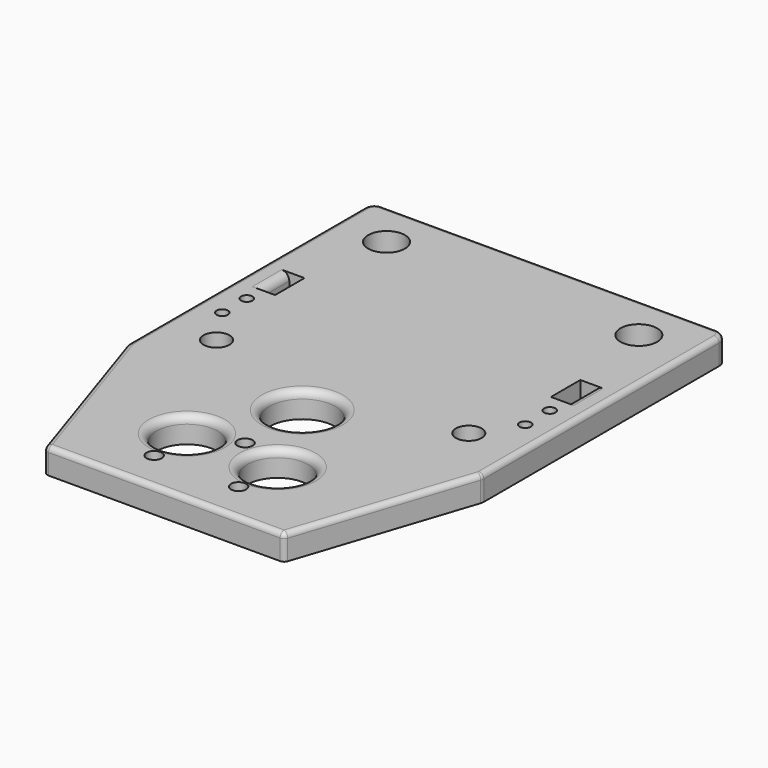
from build123d import *

# Parameters (mm, degrees)
F0_R     = 1.5
F0_R_2   = 6
F0_R_3   = 2.55
F0_R_4   = 6.5
F0_R_5   = 1.125
F0_W     = 3
F0_H     = 7.25
F0_R_6   = 3.625
F1_DEPTH = 5
F2_R     = 1.5
F3_R     = 1.5
F4_SIZE  = 1.5
F5_SIZE  = 1.5
F7_R     = 1


# Not quite as in the source:
# - a fillet or chamfer that OpenCascade refuses, or shapes differently, is made with other operations: its cross-section is extruded or revolved along the edge and cut away or added


with BuildPart() as f1:
    # F0 (on Top) → F1 (new body)
    with BuildSketch(Plane.XY):
        with BuildLine():
            Line((33, 31.9801117687), (0, 31.9801117687))
            Line((0, 31.9801117687), (-33, 31.9801117687))
            ThreePointArc((-33, 31.9801117687), (-34.4142135624, 31.3943253311), (-35, 29.9801117687))
            Line((-35, 29.9801117687), (-35, 0))
            Line((-35, 0), (-35, -28.0198882313))
            ThreePointArc((-35, -28.0198882313), (-34.9746687808, -28.337194402), (-34.899316794, -28.6464628206))
            Line((-34.899316794, -28.6464628206), (-23.5597051086, -63.0198882313))
            Line((-23.5597051086, -63.0198882313), (0, -63.0198882313))
            Line((0, -63.0198882313), (23.5597051086, -63.0198882313))
            Line((23.5597051086, -63.0198882313), (34.899316794, -28.6464628206))
            ThreePointArc((34.899316794, -28.6464628206), (34.9746687808, -28.337194402), (35, -28.0198882313))
            Line((35, -28.0198882313), (35, 0))
            Line((35, 0), (35, 29.9801117687))
            ThreePointArc((35, 29.9801117687), (34.4142135624, 31.3943253311), (33, 31.9801117687))
        make_face()
        with Locations((-8.325, -55.1198882313)):
            Circle(F0_R, mode=Mode.SUBTRACT)
        with Locations((-8.95, -46.2698882313)):
            Circle(F0_R_2, mode=Mode.SUBTRACT)
        with Locations((-24.875, -19.0698882313)):
            Circle(F0_R_3, mode=Mode.SUBTRACT)
        with Locations((8.325, -55.1198882313)):
            Circle(F0_R, mode=Mode.SUBTRACT)
        with Locations((0, -43.1198882313)):
            Circle(F0_R, mode=Mode.SUBTRACT)
        with Locations((8.95, -46.2698882313)):
            Circle(F0_R_2, mode=Mode.SUBTRACT)
        with Locations((0, -29.0198882313)):
            Circle(F0_R_4, mode=Mode.SUBTRACT)
        with Locations((24.875, -19.0698882313)):
            Circle(F0_R_3, mode=Mode.SUBTRACT)
        with Locations((-29.875, -11.3948882313)):
            Circle(F0_R_5, mode=Mode.SUBTRACT)
        with Locations((-29.875, -5.3448882313)):
            Circle(F0_R_5, mode=Mode.SUBTRACT)
        with Locations((-28.7, 1.9051117687)):
            Rectangle(F0_W, F0_H, mode=Mode.SUBTRACT)
        with Locations((-24.875, 22.8551117687)):
            Circle(F0_R_6, mode=Mode.SUBTRACT)
        with Locations((29.875, -11.3948882313)):
            Circle(F0_R_5, mode=Mode.SUBTRACT)
        with Locations((29.875, -5.3448882313)):
            Circle(F0_R_5, mode=Mode.SUBTRACT)
        with Locations((28.7, 1.9051117687)):
            Rectangle(F0_W, F0_H, mode=Mode.SUBTRACT)
        with Locations((24.875, 22.8551117687)):
            Circle(F0_R_6, mode=Mode.SUBTRACT)
    extrude(amount=F1_DEPTH)

    # F2
    f2_edges = [f1.edges().sort_by_distance(p)[0] for p in [
        (30.2, 1.905112, 5),
    ]]
    fillet(f2_edges, radius=F2_R)

    # F3
    f3_edges = [f1.edges().sort_by_distance(p)[0] for p in [
        (-30.2, 1.905112, 5),
    ]]
    fillet(f3_edges, radius=F3_R)

    # F4
    f4_edges = [f1.edges().sort_by_distance(p)[0] for p in [
        (30.2, 1.905112, 0),
    ]]
    chamfer(f4_edges, length=F4_SIZE)

    # F5
    f5_edges = [f1.edges().sort_by_distance(p)[0] for p in [
        (-30.2, 1.905112, 0),
    ]]
    chamfer(f5_edges, length=F5_SIZE)

    # F6: fillet of radius 1.5 on 3 edges, made by hand

    # F6_s1 → F6_t2 (revolve, cut)
    with BuildSketch(Plane.XZ.offset(29.0198882313)):
        with BuildLine():
            ThreePointArc((6.5, 3.5), (6.9393398282, 4.5606601718), (8, 5))
            Line((8, 5), (6.5, 5))
            Line((6.5, 5), (6.5, 3.5))
        make_face()
    revolve(axis=Axis((0, -29.0198882313, 5), (0, 0, 1)), mode=Mode.SUBTRACT)

    # F6_s3 → F6_t4 (revolve, cut)
    with BuildSketch(Plane.XZ.offset(46.2698882313)):
        with BuildLine():
            ThreePointArc((-2.95, 3.5), (-2.5106601718, 4.5606601718), (-1.45, 5))
            Line((-1.45, 5), (-2.95, 5))
            Line((-2.95, 5), (-2.95, 3.5))
        make_face()
    revolve(axis=Axis((-8.95, -46.2698882313, 5), (0, 0, 1)), mode=Mode.SUBTRACT)

    # F6_s5 → F6_t6 (revolve, cut)
    with BuildSketch(Plane.XZ.offset(46.2698882313)):
        with BuildLine():
            ThreePointArc((14.95, 3.5), (15.3893398282, 4.5606601718), (16.45, 5))
            Line((16.45, 5), (14.95, 5))
            Line((14.95, 5), (14.95, 3.5))
        make_face()
    revolve(axis=Axis((8.95, -46.2698882313, 5), (0, 0, 1)), mode=Mode.SUBTRACT)

    # F7
    f7_edges = [f1.edges().sort_by_distance(p)[0] for p in [
        (29.229511, -45.833176, 5),
        (0, -63.019888, 5),
        (23.559705, -63.019888, 2.5),
        (-23.559705, -63.019888, 2.5),
        (34.974669, -28.337194, 5),
        (-34.974669, -28.337194, 5),
        (0, 31.980112, 5),
        (-34.414214, 31.394325, 5),
        (-35, 0.980112, 5),
        (-29.229511, -45.833176, 5),
        (35, 0.980112, 5),
        (34.414214, 31.394325, 5),
    ]]
    fillet(f7_edges, radius=F7_R)


solid = f1.part
